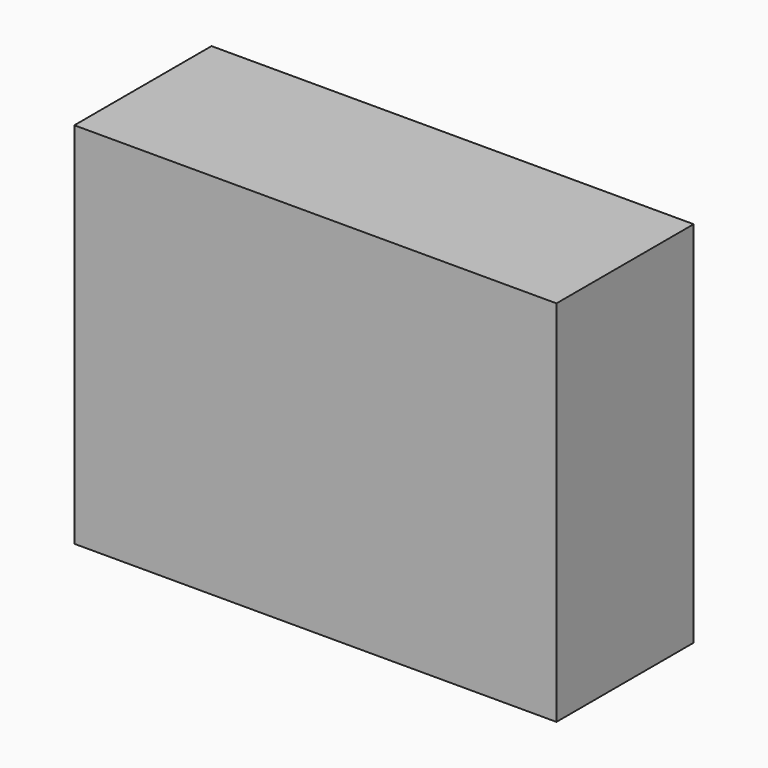
from build123d import *

# Parameters (mm, degrees)
F0_W     = 71.4176669717
F0_H     = 54.5815601945
F1_DEPTH = 25.4


# Not quite as in the source:
# - the program builds the solid bodies; features that only make, move or delete a surface that nothing else refers to are left out


with BuildPart() as f1:
    # F0 (on Front) → F1 (new body)
    with BuildSketch(Plane.XZ):
        with Locations((0.3310590982, 6.7904144526)):
            Rectangle(F0_W, F0_H)
    extrude(amount=F1_DEPTH)


solid = f1.part
